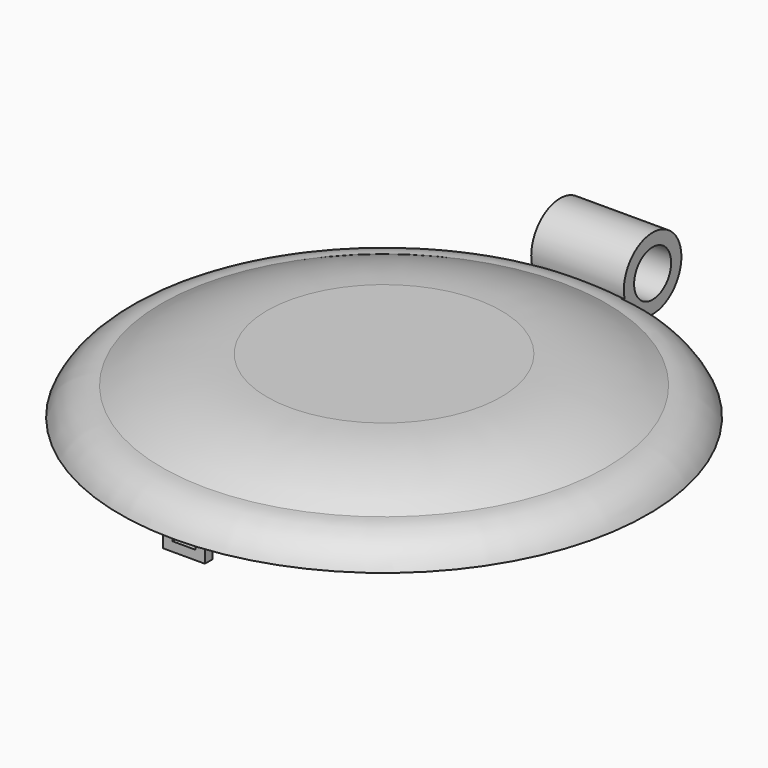
from build123d import *

# Parameters (mm, degrees)
F0_R      = 28.5
F0_R_2    = 22.5
F1_DEPTH  = 3
F3_ANGLE  = -90
F4_W      = 1.5
F4_H      = 3
F7_START  = 26
F7_DEPTH  = 1
F8_R      = 3.88474
F8_R_2    = 2.5
F9_DEPTH  = 5
F10_START = -5
F8_R_3    = 4.38474
F10_DEPTH = 3.5
F11_START = 5
F11_DEPTH = 3.5
F12_START = 24
F4_W_2    = 2.5
F4_H_2    = 1
F12_DEPTH = 3


# Not quite as in the source:
# - a fillet or chamfer that OpenCascade refuses, or shapes differently, is made with other operations: its cross-section is extruded or revolved along the edge and cut away or added


with BuildPart() as f1:
    # F0 (on Top) → F1 (new body)
    with BuildSketch(Plane.XY):
        Circle(F0_R)
        Circle(F0_R_2, mode=Mode.SUBTRACT)
    extrude(amount=F1_DEPTH)

    # F2: fillet of radius 5 on 1 edges, made by hand

    # F2_s1 → F2_t2 (revolve, cut)
    with BuildSketch(Plane.XZ):
        with BuildLine():
            ThreePointArc((28.5, 0), (26.6560370926, 2.1833001327), (23.917424305, 3))
            Line((23.917424305, 3), (28.5, 3))
            Line((28.5, 3), (28.5, 0))
        make_face()
    revolve(axis=Axis((0, 0, 3), (0, 0, 1)), mode=Mode.SUBTRACT)


with BuildPart() as f1_1:
    # F3: moved
    add(f1.part.rotate(Axis((0, 0, -1.9999999998), (0, 0, 1)), F3_ANGLE))

    # F4 (on Front) → F7 (join)
    with BuildSketch(Plane.XZ.offset(F7_START)):
        Polygon((1.25, -1.25), (-1.25, -1.25), (-1.25, 0), (-2.25, 0), (-2.25, -2.25), (2.25, -2.25), (2.25, 0), (1.25, 0), align=None)
    extrude(amount=F7_DEPTH)

    # F8 (on Right) → F9 (join, symmetric)
    with BuildSketch(Plane.YZ):
        with Locations((30, 3.07777)):
            Circle(F8_R)
        with Locations((30, 3.07777)):
            Circle(F8_R_2, mode=Mode.SUBTRACT)
    extrude(amount=F9_DEPTH, both=True)

    # F8 (on Right) → F10 (cut)
    with BuildSketch(Plane.YZ.offset(F10_START)):
        with Locations((30, 3.07777)):
            Circle(F8_R_3)
        with Locations((30, 3.07777)):
            Circle(F8_R, mode=Mode.SUBTRACT)
        with Locations((30, 3.07777)):
            Circle(F8_R)
        with Locations((30, 3.07777)):
            Circle(F8_R_2, mode=Mode.SUBTRACT)
    extrude(amount=-F10_DEPTH, mode=Mode.SUBTRACT)

    # F8 (on Right) → F11 (cut)
    with BuildSketch(Plane.YZ.offset(F11_START)):
        with Locations((30, 3.07777)):
            Circle(F8_R_3)
        with Locations((30, 3.07777)):
            Circle(F8_R, mode=Mode.SUBTRACT)
        with Locations((30, 3.07777)):
            Circle(F8_R)
        with Locations((30, 3.07777)):
            Circle(F8_R_2, mode=Mode.SUBTRACT)
    extrude(amount=F11_DEPTH, mode=Mode.SUBTRACT)

    # F4 (on Front) → F12 (cut)
    with BuildSketch(Plane.XZ.offset(F12_START)):
        with Locations((0, 0.5)):
            Rectangle(F4_W_2, F4_H_2)
    extrude(amount=F12_DEPTH, mode=Mode.SUBTRACT)


with BuildPart() as f5:
    # F4 (on Front) → F5 (revolve)
    with BuildSketch(Plane.XZ):
        Polygon((0, 4), (0, 6), (-22.5, 6), (-22.5, 3), align=None)
        with Locations((-23.25, 4.5)):
            Rectangle(F4_W, F4_H)
        Polygon((-22.5, 0), (0, 4), (-22.5, 3), align=None)
    revolve(axis=Axis((0, 0, 5), (0, 0, -1)))

    # F6: fillet of radius 23 on 1 edges, made by hand

    # F6_s1 → F6_t2 (revolve, cut)
    with BuildSketch(Plane.XZ):
        with BuildLine():
            ThreePointArc((-12.6421833084, 6), (-18.5158533706, 5.2373559579), (-24, 3))
            Line((-24, 3), (-24, 6))
            Line((-24, 6), (-12.6421833084, 6))
        make_face()
    revolve(axis=Axis((0, 0, 6), (0, 0, -1)), mode=Mode.SUBTRACT)


solid = Compound([f1_1.part, f5.part])
